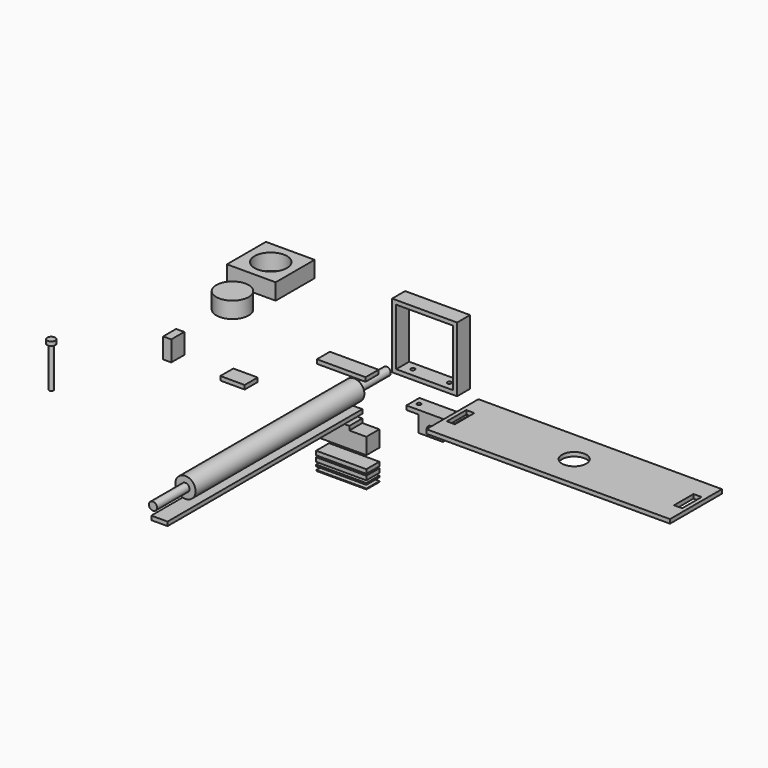
from build123d import *

# Parameters (mm, degrees)
F0_R      = 5
F1_DEPTH  = 20
F0_W      = 60
F0_H      = 5
F0_W_2    = 80
F0_H_2    = 80
F0_W_3    = 70
F0_H_3    = 70
F0_W_4    = 61.861140081
F0_H_4    = 1
F0_H_5    = 2
F0_R_2    = 12.5
F2_DEPTH  = 260
F3_R      = 5
F4_DEPTH  = 50
F5_DEPTH  = 300
F6_R      = 2.5
F7_DEPTH  = 25
F9_R      = 2.5
F8_R      = 2.5
F10_DEPTH = 25
F14_R     = 5
F15_DEPTH = 50
F16_W     = 300
F16_H     = 5
F17_DEPTH = 80
F19_R     = 20
F20_DEPTH = 20
F19_W     = 60
F19_H     = 60
F21_DEPTH = 20
F18_W     = 10
F18_H     = 30
F18_R     = 15
F22_DEPTH = 129.4251411048
F18_H_2   = 20
F23_DEPTH = 25
F18_W_2   = 30
F24_DEPTH = 5
F13_R     = 2.5
F25_DEPTH = 5
F26_R     = 5
F27_DEPTH = 5
F28_R     = 2.5
F29_DEPTH = 50


# Not quite as in the source:
# - a feature of the source that left no trace in its solid (it failed there, or was rolled back) is left out
# - a feature names something its author has since deleted; it is built from what else it names


with BuildPart() as f1:
    # F0 (on Front) → F1 (new body)
    with BuildSketch(Plane.XZ):
        Polygon((95.2936565876, -7.5), (110.2936565876, -7.5), (125.2936565876, -7.5), (125.2936565876, 12.5), (140.2936565876, 12.5), (140.2936565876, 17.5), (110.2936565876, 17.5), (80.2936565876, 17.5), (80.2936565876, 12.5), (95.2936565876, 12.5), align=None)
        with Locations((110.2936565876, 0)):
            Circle(F0_R, mode=Mode.SUBTRACT)
    extrude(amount=F1_DEPTH)

    # F9 (on face) + F8 (on face) → F10 (cut)
    with BuildSketch(Plane(origin=(0, 0, 12.5), x_dir=(1, 0, 0), z_dir=(0, 0, -1))):
        with Locations((87.7936565876, 10)):
            Circle(F9_R)
    with BuildSketch(Plane(origin=(0, 0, 12.5), x_dir=(1, 0, 0), z_dir=(0, 0, -1))):
        with Locations((132.7936565876, 10)):
            Circle(F8_R)
    extrude(amount=-F10_DEPTH, mode=Mode.SUBTRACT)


with BuildPart() as f1b:
    # F0 (on Front) → F1, piece 2 (new body)
    with BuildSketch(Plane.XZ):
        with Locations((0, 29.2427036911)):
            Rectangle(F0_W, F0_H)
    extrude(amount=F1_DEPTH)


with BuildPart() as f1c:
    # F0 (on Front) → F1, piece 3 (new body)
    with BuildSketch(Plane.XZ):
        Polygon((10, -27.5771580637), (0, -27.5771580637), (-10, -27.5771580637), (-10, -32.5771580637), (-10.9305700405, -32.5771580637), (-30.9305700405, -32.5771580637), (-30.9305700405, -52.5771580637), (0, -52.5771580637), (30.9305700405, -52.5771580637), (30.9305700405, -32.5771580637), (10.9305700405, -32.5771580637), (10, -32.5771580637), align=None)
    extrude(amount=F1_DEPTH)

    # F6 (on face) → F7 (cut)
    with BuildSketch(Plane.XY.offset(-32.5771580637)):
        with Locations((-20, -10)):
            Circle(F6_R)
    extrude(amount=-F7_DEPTH, mode=Mode.SUBTRACT)


with BuildPart() as f1d:
    # F0 (on Front) → F1, piece 4 (new body)
    with BuildSketch(Plane.XZ):
        with Locations((102.7326732874, 87.7068325877)):
            Rectangle(F0_W_2, F0_H_2)
        with Locations((102.7326732874, 87.7068325877)):
            Rectangle(F0_W_3, F0_H_3, mode=Mode.SUBTRACT)
    extrude(amount=F1_DEPTH)

    # F13 (on face) → F25 (cut, through all)
    with BuildSketch(Plane(origin=(0, 0, 47.7068325877), x_dir=(1, 0, 0), z_dir=(0, 0, -1))):
        with Locations((125.2326732874, 10)):
            Circle(F13_R)
        with Locations((80.2326732874, 10)):
            Circle(F13_R)
    extrude(amount=-F25_DEPTH, mode=Mode.SUBTRACT)


with BuildPart() as f1e:
    # F0 (on Front) → F1, piece 5 (new body)
    with BuildSketch(Plane.XZ):
        with Locations((0, -77.355325222)):
            Rectangle(F0_W_4, F0_H)
    extrude(amount=F1_DEPTH)


with BuildPart() as f1f:
    # F0 (on Front) → F1, piece 6 (new body)
    with BuildSketch(Plane.XZ):
        with Locations((0.1928325291, -89.1451310813)):
            Rectangle(F0_W_4, F0_H_4)
    extrude(amount=F1_DEPTH)


with BuildPart() as f1g:
    # F0 (on Front) → F1, piece 7 (new body)
    with BuildSketch(Plane.XZ):
        with Locations((0, -83.756296128)):
            Rectangle(F0_W_4, F0_H_5)
    extrude(amount=F1_DEPTH)


with BuildPart() as f1h:
    # F0 (on Front) → F1, piece 8 (new body)
    with BuildSketch(Plane.XZ):
        with Locations((0, -70.2389810979)):
            Rectangle(F0_W_4, F0_H)
    extrude(amount=F1_DEPTH)


with BuildPart() as f2:
    # F0 (on Front) → F2 (new body)
    with BuildSketch(Plane.XZ):
        Circle(F0_R_2)
    extrude(amount=F2_DEPTH)

    # F3 (on face) → F4 (join)
    with BuildSketch(Plane.XZ.offset(260)):
        Circle(F3_R)
    extrude(amount=F4_DEPTH)

    # F14 (on face) → F15 (join)
    with BuildSketch(Plane(origin=(0, 0, 0), x_dir=(-1, 0, 0), z_dir=(0, 1, 0))):
        Circle(F14_R)
    extrude(amount=F15_DEPTH)


with BuildPart() as f5:
    # F0 (on Front) → F5 (new body)
    with BuildSketch(Plane.XZ):
        Polygon((-10, -22.5167013705), (0, -22.5167013705), (10, -22.5167013705), (10, -17.5167013705), (0, -17.5167013705), (-10, -17.5167013705), align=None)
    extrude(amount=F5_DEPTH)


with BuildPart() as f17:
    # F16 (on Front) → F17 (new body)
    with BuildSketch(Plane.XZ):
        with Locations((303.0256081372, 37.2790100235)):
            Rectangle(F16_W, F16_H)
    extrude(amount=F17_DEPTH)

    # F18 (on face) → F22 (cut, through all)
    with BuildSketch(Plane.XY.offset(39.7790100235)):
        with Locations((163.0256081372, -40)):
            Rectangle(F18_W, F18_H)
        with Locations((443.0256081372, -40)):
            Rectangle(F18_W, F18_H)
        with Locations((303.0256081372, -40)):
            Circle(F18_R)
    extrude(amount=-F22_DEPTH, mode=Mode.SUBTRACT)


with BuildPart() as f20:
    # F19 (on Top) → F20 (new body)
    with BuildSketch(Plane.XY):
        with Locations((-196.2528675795, 57.794149965)):
            Circle(F19_R)
    extrude(amount=F20_DEPTH)


with BuildPart() as f21:
    # F19 (on Top) → F21 (new body)
    with BuildSketch(Plane.XY):
        with Locations((-205.1943850517, 127.9719012976)):
            Rectangle(F19_W, F19_H)
        with Locations((-205.1943850517, 127.9719012976)):
            Circle(F19_R, mode=Mode.SUBTRACT)
    extrude(amount=F21_DEPTH)


with BuildPart() as f23:
    # F18 (on face) → F23 (new body)
    with BuildSketch(Plane.XY.offset(39.7790100235)):
        with Locations((-130.5344802141, -114.8494374752)):
            Rectangle(F18_W, F18_H_2)
    extrude(amount=F23_DEPTH)


with BuildPart() as f24:
    # F18 (on face) → F24 (new body)
    with BuildSketch(Plane.XY.offset(39.7790100235)):
        with Locations((-50.0688782334, -114.8494374752)):
            Rectangle(F18_W_2, F18_H_2)
    extrude(amount=F24_DEPTH)


with BuildPart() as f27:
    # F26 (on Top) → F27 (new body)
    with BuildSketch(Plane.XY):
        with Locations((-287.8777384163, -106.7102653366)):
            Circle(F26_R)
    extrude(amount=F27_DEPTH)

    # F28 (on face) → F29 (join)
    with BuildSketch(Plane.XY):
        with Locations((-287.7346277237, -106.8533882499)):
            Circle(F28_R)
    extrude(amount=-F29_DEPTH)


solid = Compound([f1.part, f1b.part, f1c.part, f1d.part, f1e.part, f1f.part, f1g.part, f1h.part, f2.part, f5.part, f17.part, f20.part, f21.part, f23.part, f24.part, f27.part])
